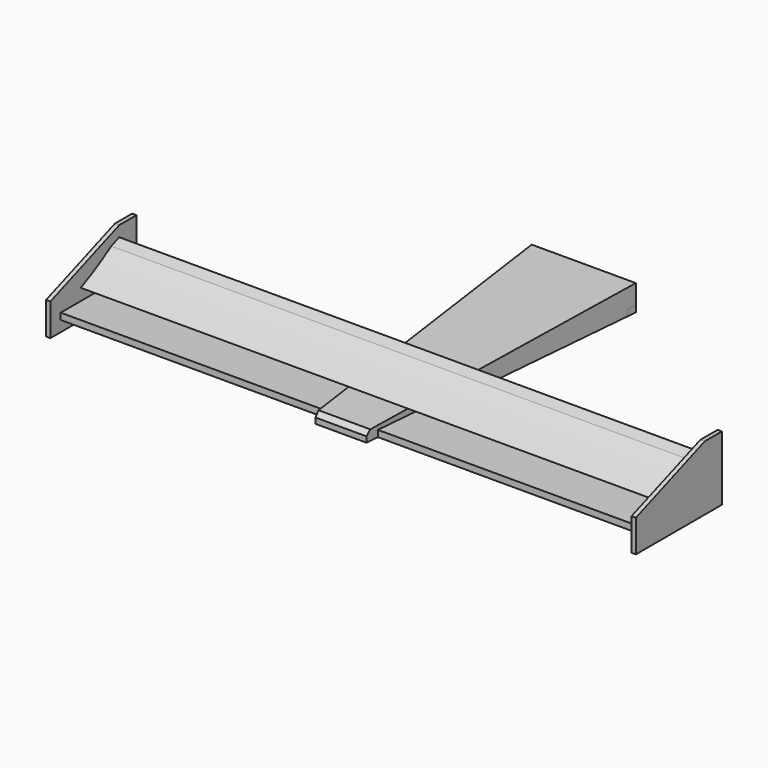
from build123d import *

# Parameters (mm, degrees)
F1_DEPTH       = 15
F2_W           = 150
F2_H           = 15
F3_DEPTH       = 10
F4_W           = 250
F4_H           = 75
F4_W_2         = 150
F4_H_2         = 15
F5_DEPTH       = 10
F7_DEPTH       = 45
F9_DEPTH       = 1350
F11_DEPTH      = 675
F11_DEPTH_BACK = 675
F12_SIZE       = 10


# Not quite as in the source:
# - an extrude ends at something that could not be found from the text; its depth is read off the source's solid


with BuildPart() as f1:
    # F0 (on Top) → F1 (new body)
    with BuildSketch(Plane.XY):
        Polygon((-61.8767004711, -675), (-75, -525), (-675, -525), (-675, -675), align=None)
        Polygon((0, -525), (0, 0), (-120.9315483511, 0), (-119.0390060495, -21.6318574922), (-75, -525), align=None)
        Polygon((120.9315483511, 0), (0, 0), (0, -525), (75, -525), (119.0390060495, -21.6318574922), align=None)
        Polygon((0, -705), (0, -525), (-75, -525), (-61.8767004711, -675), (-59.2520405653, -705), align=None)
        Polygon((75, -525), (0, -525), (0, -705), (59.2520405653, -705), (61.8767004711, -675), align=None)
        Polygon((675, -525), (75, -525), (61.8767004711, -675), (675, -675), align=None)
    extrude(amount=F1_DEPTH)

    # F2 (on face) → F3 (join)
    with BuildSketch(Plane.YZ.offset(675)):
        Polygon((-505, 125), (-705, 50), (-455, 50), (-455, 125), align=None)
        Polygon((-705, 50), (-705, 0), (-705, -25), (-455, -25), (-455, 50), align=None)
        with Locations((-600, 7.5)):
            Rectangle(F2_W, F2_H, mode=Mode.SUBTRACT)
        with Locations((-600, 7.5)):
            Rectangle(F2_W, F2_H)
    extrude(amount=F3_DEPTH)

    # F6 (on face) → F7 (join)
    with BuildSketch(Plane.XY.offset(15)):
        Polygon((120.9315483511, 0), (-120.9315483511, 0), (-59.2520405653, -705), (59.2520405653, -705), align=None)
    extrude(amount=F7_DEPTH)

    # F10 (on Right) → F11 (cut, two sides)
    with BuildSketch(Plane.YZ) as f11_sk:
        Polygon((-826.1129958937, 16.7052524484), (0, 60), (-829.8766534977, 88.5201176353), align=None)
    extrude(amount=F11_DEPTH, mode=Mode.SUBTRACT)
    extrude(f11_sk.sketch, amount=-F11_DEPTH_BACK, mode=Mode.SUBTRACT)

    # F12
    f12_edges = [f1.edges().sort_by_distance(p)[0] for p in [
        (0, -705, 23.052516),
    ]]
    chamfer(f12_edges, length=F12_SIZE)


with BuildPart() as f5:
    # F4 (on face) → F5 (new body)
    with BuildSketch(Plane(origin=(-675, 0, 0), x_dir=(0, -1, 0), z_dir=(-1, 0, 0))):
        Polygon((455, 125), (455, 50), (705, 50), (505, 125), align=None)
        with Locations((580, 12.5)):
            Rectangle(F4_W, F4_H)
        with Locations((600, 7.5)):
            Rectangle(F4_W_2, F4_H_2, mode=Mode.SUBTRACT)
        with Locations((600, 7.5)):
            Rectangle(F4_W_2, F4_H_2)
    extrude(amount=F5_DEPTH)


with BuildPart() as f9:
    # F8 (on face) → F9 (new body, through all)
    with BuildSketch(Plane(origin=(675, 0, 0), x_dir=(0, -1, 0), z_dir=(-1, 0, 0))):
        with BuildLine():
            Line((528.4082294392, 91.3629019553), (505, 100.140987995))
            Line((505, 100.140987995), (499.7331483762, 86.0960503315))
            Line((499.7331483762, 86.0960503315), (616.7742955723, 42.2056201329))
            ThreePointArc((616.7742955723, 42.2056201329), (571.5538504506, 64.9193893734), (528.4082294392, 91.3629019553))
        make_face()
    extrude(amount=F9_DEPTH)


solid = Compound([f1.part, f5.part, f9.part])
